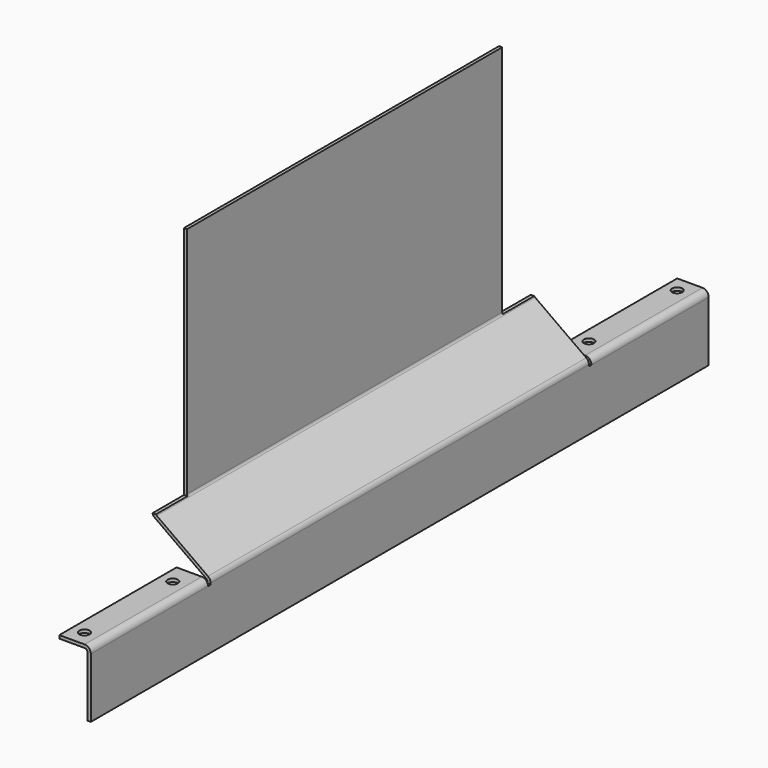
from build123d import *

# Parameters (mm, degrees)
F1_DEPTH  = 150
F3_DEPTH  = 95
F4_W      = 2
F4_H      = 56
F6_DEPTH  = 25
F5_W      = 55.4491758279
F5_H      = 188.3780552482
F7_DEPTH  = 50
F8_R      = 2
F9_R      = 4
F10_R     = 3.25
F11_DEPTH = 25


# Not quite as in the source:
# - a pattern or mirror of a feature is missing from the dataset's text; its kind, count and spacing are read off the source's solid


with BuildPart() as f1:
    # F0 (on Front) → F1 (new body, symmetric)
    with BuildSketch(Plane.XZ):
        Polygon((1, -26), (1, -66), (3, -66), (3, -24.9707642094), (-32, 0.0292357906), (-32, 149), (-34, 149), (-34, -1), align=None)
    extrude(amount=F1_DEPTH, both=True)

    # F2 (on face) → F3 (join)
    with BuildSketch(Plane.XZ.offset(150)):
        Polygon((1.6409301068, -24), (3, -24.9707642094), (3, -24), align=None)
        Polygon((-17, -26), (1, -26), (-1.8, -24), (-17, -24), align=None)
        Polygon((1, -27.0292357906), (1, -66), (3, -66), (3, -24.9707642094), (1.6409301068, -24), (-1.8, -24), (1, -26), align=None)
    f3 = extrude(amount=F3_DEPTH)

    # F3_copies: F3 across plane
    add(f3.mirror(Plane.ZX))

    # F4 (on face) → F6 (cut)
    with BuildSketch(Plane.YZ.offset(3)):
        with Locations((-151, 0)):
            Rectangle(F4_W, F4_H)
        with Locations((151, 0)):
            Rectangle(F4_W, F4_H)
    extrude(amount=-F6_DEPTH, mode=Mode.SUBTRACT)

    # F5 (on face) → F7 (cut)
    with BuildSketch(Plane.YZ.offset(3)):
        with Locations((152.724587914, 94.1890276241)):
            Rectangle(F5_W, F5_H)
        with Locations((-152.724587914, 94.1890276241)):
            Rectangle(F5_W, F5_H)
    extrude(amount=-F7_DEPTH, mode=Mode.SUBTRACT)

    # F8
    f8_edges = [f1.edges().sort_by_distance(p)[0] for p in [
        (-32, 0, 0.029236),
        (1, -198.5, -26),
        (1, 0, -26),
        (1, 198.5, -26),
    ]]
    fillet(f8_edges, radius=F8_R)

    # F9
    f9_edges = [f1.edges().sort_by_distance(p)[0] for p in [
        (3, -198.5, -24),
        (3, 0, -24.970764),
        (-34, 0, -1),
        (3, 198.5, -24),
    ]]
    fillet(f9_edges, radius=F9_R)

    # F10 (on face) → F11 (cut)
    with BuildSketch(Plane.XY.offset(-24)):
        with Locations((-9, 235)):
            Circle(F10_R)
        with Locations((-9, 165)):
            Circle(F10_R)
        with Locations((-9, -165)):
            Circle(F10_R)
        with Locations((-9, -235)):
            Circle(F10_R)
    extrude(amount=-F11_DEPTH, mode=Mode.SUBTRACT)


solid = f1.part
